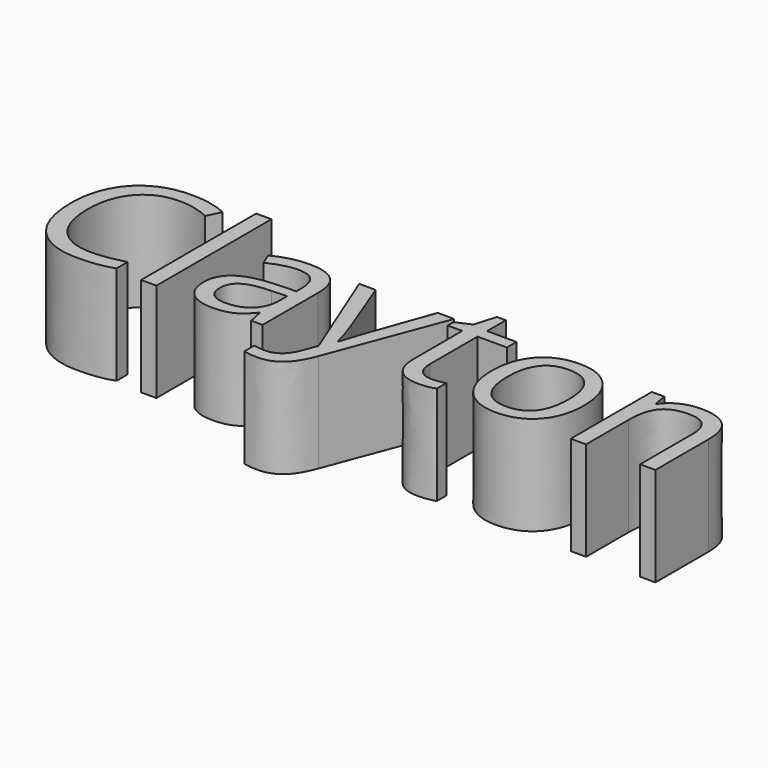
from build123d import *

# Parameters (mm, degrees)
F0_TEXT_SIZE = 97.1305158196
F1_DEPTH     = 50.8


# Not quite as in the source:
# - Text() gives the source's letters only with a copy of the font that has no kerning and outlines rounded to 1/6400 em; it was checked with that copy


with BuildPart() as f1:
    # F0 (on Top) → F1 (new body)
    with BuildSketch(Plane.XY):
        with Locations((-139.4794285297, -81.9781571627)):
            Text('Clayton', F0_TEXT_SIZE, font='Open Sans', text_align=(TextAlign.LEFT, TextAlign.BOTTOM))
    extrude(amount=F1_DEPTH)


solid = f1.part
